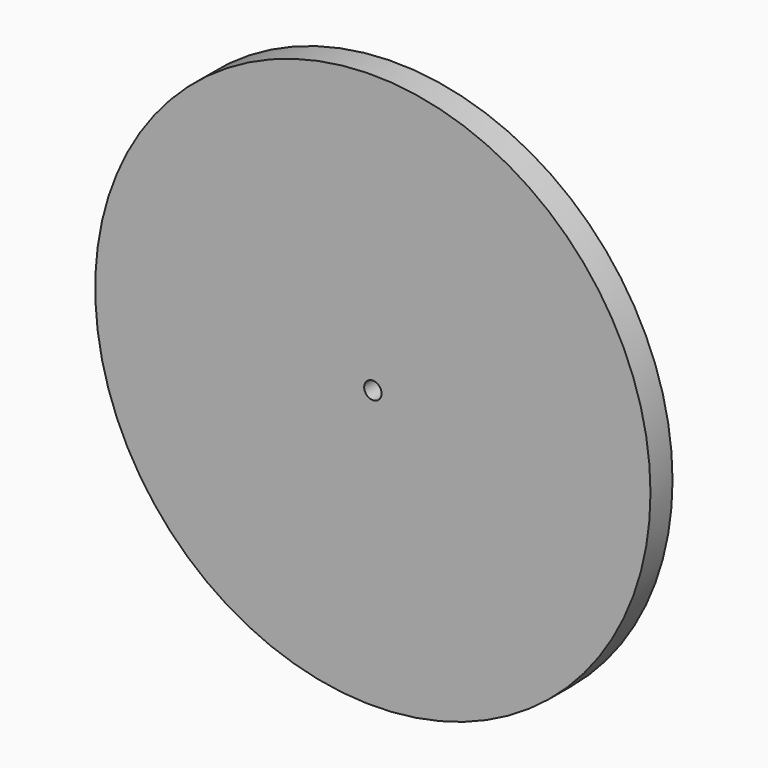
from build123d import *

# Parameters (mm, degrees)
F0_R     = 48
F0_R_2   = 1.5
F1_DEPTH = 4.7625


# Not quite as in the source:
# - a feature names something its author has since deleted; it is built from what else it names


with BuildPart() as f1:
    # F0 (on Front) → F1 (new body)
    with BuildSketch(Plane.XZ):
        with Locations((-34.7213223577, 19.0212465823)):
            Circle(F0_R)
        with Locations((-34.7213223577, 19.0212465823)):
            Circle(F0_R_2, mode=Mode.SUBTRACT)
    extrude(amount=F1_DEPTH)


solid = f1.part
